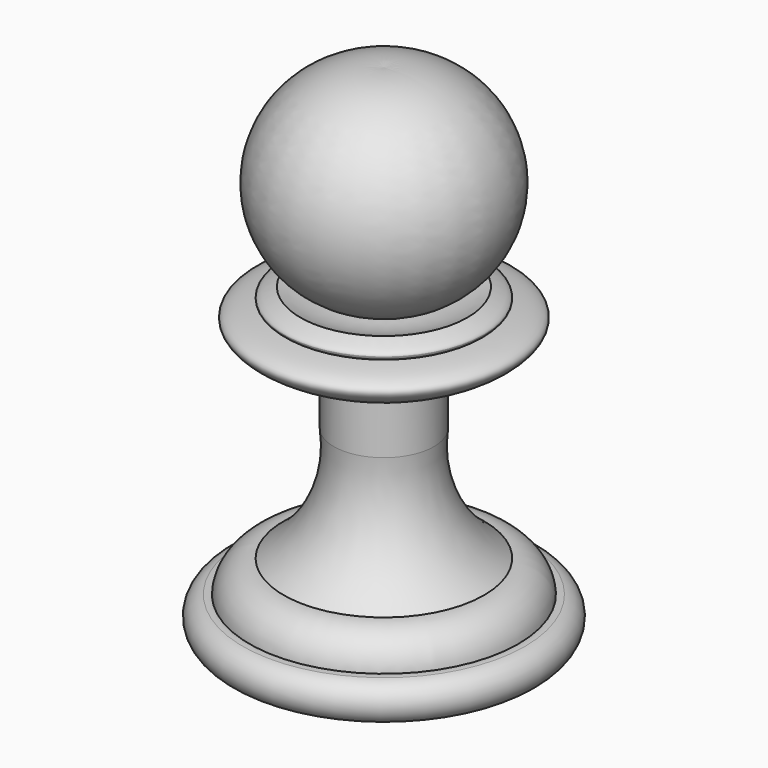
from build123d import *


with BuildPart() as f1:
    # F0 (on Front) → F1 (revolve)
    with BuildSketch(Plane.XZ):
        Polygon((0, 4.6565216035), (0, 2.2227435741), (11.817666702, 2.2227435741), (11.817666702, 5.5569853109), (0, 5.5569853109), align=None)
        with BuildLine():
            Line((11.817666702, 5.5569853109), (11.817666702, 2.2227435741))
            Line((11.817666702, 2.2227435741), (12.4022987136, 2.2227435741))
            ThreePointArc((12.4022987136, 2.2227435741), (13.8025371787, 3.8898644425), (12.4022987136, 5.5569853109))
            Line((12.4022987136, 5.5569853109), (11.817666702, 5.5569853109))
        make_face()
        with BuildLine():
            Line((12.4022987136, 2.2227435741), (11.817666702, 2.2227435741))
            ThreePointArc((11.817666702, 2.2227435741), (12.1099827078, 2.1973099715), (12.4022987136, 2.2227435741))
        make_face()
        with BuildLine():
            Line((0, 8.3557413891), (0, 5.5569853109))
            Line((0, 5.5569853109), (11.817666702, 5.5569853109))
            ThreePointArc((11.817666702, 5.5569853109), (10.8664849347, 7.5476316743), (8.8135898113, 8.3557413891))
            Line((8.8135898113, 8.3557413891), (0, 8.3557413891))
        make_face()
        with BuildLine():
            ThreePointArc((12.4022987136, 5.5569853109), (12.1099827078, 5.5824189134), (11.817666702, 5.5569853109))
            Line((11.817666702, 5.5569853109), (12.4022987136, 5.5569853109))
        make_face()
        with BuildLine():
            Line((0, 18.428416457), (0, 8.3557413891))
            Line((0, 8.3557413891), (8.8135898113, 8.3557413891))
            ThreePointArc((8.8135898113, 8.3557413891), (5.215958109, 12.7821014993), (4.4067949057, 18.428416457))
            Line((4.4067949057, 18.428416457), (4.4067949057, 23.4373846475))
            add(Edge.make_bspline(
                [(4.4067949057, 23.4373846475), (2.980322901, 23.075299344), (1.465602045, 22.810778825), (0, 22.7169202584)],
                knots=[0.5270695055, 0.5270695055, 0.5270695055, 0.5270695055, 0.6122871949, 0.6122871949, 0.6122871949, 0.6122871949], degree=3))
            Line((0, 22.7169202584), (0, 18.428416457))
        make_face()
        with BuildLine():
            Line((0, 26.2118484825), (0, 22.7169202584))
            add(Edge.make_bspline(
                [(4.4067949057, 23.4373846475), (2.980322901, 23.075299344), (1.465602045, 22.810778825), (0, 22.7169202584)],
                knots=[0.5270695055, 0.5270695055, 0.5270695055, 0.5270695055, 0.6122871949, 0.6122871949, 0.6122871949, 0.6122871949], degree=3))
            add(Edge.make_bspline(
                [(8.4766640969, 28.1302331889), (10.2132138826, 27.9217440003), (13.2094926319, 27.009468985), (8.1795813862, 24.3950413934), (4.4067949057, 23.4373846475)],
                knots=[0.1677963022, 0.1677963022, 0.1677963022, 0.1677963022, 0.3016825753, 0.5270695055, 0.5270695055, 0.5270695055, 0.5270695055], degree=3))
            add(Edge.make_bspline(
                [(8.4766640969, 28.1302331889), (7.3659928159, 27.4837834782), (3.6829964079, 26.8478159804), (0, 26.2118484825)],
                knots=[0.5116773185, 0.5116773185, 0.5116773185, 0.5116773185, 1, 1, 1, 1], degree=3))
        make_face()
        with BuildLine():
            Line((0, 28.501091525), (0, 26.2118484825))
            add(Edge.make_bspline(
                [(8.4766640969, 28.1302331889), (7.3659928159, 27.4837834782), (3.6829964079, 26.8478159804), (0, 26.2118484825)],
                knots=[0.5116773185, 0.5116773185, 0.5116773185, 0.5116773185, 1, 1, 1, 1], degree=3))
            add(Edge.make_bspline(
                [(1.4607855192, 28.4748566031), (4.1030356094, 28.4243731068), (6.6375337613, 28.3510381404), (8.4766640969, 28.1302331889)],
                knots=[0.02600117, 0.02600117, 0.02600117, 0.02600117, 0.1677963022, 0.1677963022, 0.1677963022, 0.1677963022], degree=3))
            ThreePointArc((1.4607855192, 28.4748566031), (0.7298578761, 28.4581912398), (0, 28.501091525))
        make_face()
        with BuildLine():
            add(Edge.make_bspline(
                [(1.4607855192, 28.4748566031), (4.1030356094, 28.4243731068), (6.6375337613, 28.3510381404), (8.4766640969, 28.1302331889)],
                knots=[0.02600117, 0.02600117, 0.02600117, 0.02600117, 0.1677963022, 0.1677963022, 0.1677963022, 0.1677963022], degree=3))
            add(Edge.make_bspline(
                [(8.8135898113, 28.501091525), (8.8066058004, 28.3770428825), (8.6883599805, 28.2534476314), (8.4766640969, 28.1302331889)],
                knots=[0.4186021635, 0.4186021635, 0.4186021635, 0.4186021635, 0.5116773185, 0.5116773185, 0.5116773185, 0.5116773185], degree=3))
            Line((8.8135898113, 28.501091525), (8.8135898113, 28.524566569))
            add(Edge.make_bspline(
                [(7.3526566865, 29.3778236866), (8.2135287932, 29.0918810295), (8.7977668825, 28.8070656547), (8.8135898113, 28.524566569)],
                knots=[0.2008669102, 0.2008669102, 0.2008669102, 0.2008669102, 0.4127323097, 0.4127323097, 0.4127323097, 0.4127323097], degree=3))
            ThreePointArc((7.3526566865, 29.3778236866), (5.4142100876, 28.8238626486), (3.398185771, 28.8141671216))
            ThreePointArc((3.398185771, 28.8141671216), (2.4388115043, 28.5912629325), (1.4607855192, 28.4748566031))
        make_face()
        with BuildLine():
            Line((0, 38.784313947), (0, 28.501091525))
            add(Edge.make_bspline(
                [(0, 28.501091525), (0.4881362284, 28.4926026784), (0.9762724568, 28.4841138319), (1.4607855192, 28.4748566031)],
                knots=[0, 0, 0, 0, 0.02600117, 0.02600117, 0.02600117, 0.02600117], degree=3))
            ThreePointArc((1.4607855192, 28.4748566031), (2.4388115043, 28.5912629325), (3.398185771, 28.8141671216))
            ThreePointArc((3.398185771, 28.8141671216), (4.5882717645, 29.253942465), (5.7044288291, 29.8571840683))
            ThreePointArc((5.7044288291, 29.8571840683), (9.3708930125, 40.3608451965), (0, 46.3571958244))
            Line((0, 46.3571958244), (0, 38.784313947))
        make_face()
        with BuildLine():
            add(Edge.make_bspline(
                [(0, 28.501091525), (0.4881362284, 28.4926026784), (0.9762724568, 28.4841138319), (1.4607855192, 28.4748566031)],
                knots=[0, 0, 0, 0, 0.02600117, 0.02600117, 0.02600117, 0.02600117], degree=3))
            ThreePointArc((0, 28.501091525), (0.7298578761, 28.4581912398), (1.4607855192, 28.4748566031))
        make_face()
        with BuildLine():
            Line((8.8135898113, 28.524566569), (8.8135898113, 28.501091525))
            add(Edge.make_bspline(
                [(8.8135898113, 28.524566569), (8.8140281948, 28.5167397679), (8.8140302632, 28.5089147448), (8.8135898113, 28.501091525)],
                knots=[0.4127323097, 0.4127323097, 0.4127323097, 0.4127323097, 0.4186021635, 0.4186021635, 0.4186021635, 0.4186021635], degree=3))
        make_face()
    revolve(axis=Axis((0, 0, 23.464753991), (0, 0, -1)))


solid = f1.part
